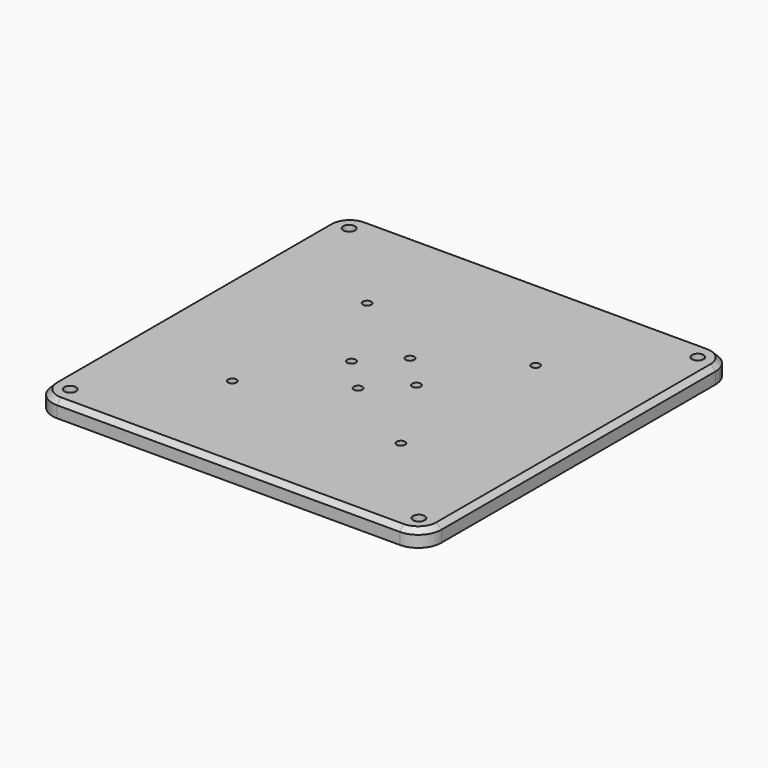
from build123d import *

# Parameters (mm, degrees)
F0_W           = 300
F0_H           = 300
F1_DEPTH       = 12.7
F2_R           = 17.78
F3_SIZE        = 3.81
F5_D           = 9
F7_D           = 6.5278
F9_D           = 6.6
F9_CSINK_D     = 13.44
F9_CSINK_ANGLE = 90


with BuildPart() as f1:
    # F0 (on Top) → F1 (new body)
    with BuildSketch(Plane.XY):
        Rectangle(F0_W, F0_H)
    extrude(amount=F1_DEPTH)

    # F2
    f2_edges = [f1.edges().sort_by_distance(p)[0] for p in [
        (-150, -150, 6.35),
        (150, -150, 6.35),
        (150, 150, 6.35),
        (-150, 150, 6.35),
    ]]
    fillet(f2_edges, radius=F2_R)

    # F3
    f3_edges = [f1.edges().sort_by_distance(p)[0] for p in [
        (-150, 0, 12.7),
        (0, 150, 12.7),
        (150, 0, 12.7),
        (0, -150, 12.7),
        (144.792359, -144.792359, 12.7),
        (144.792359, 144.792359, 12.7),
        (-144.792359, -144.792359, 12.7),
        (-144.792359, 144.792359, 12.7),
    ]]
    chamfer(f3_edges, length=F3_SIZE)

    # F5 (through all)
    with Locations(Plane(origin=(0, 0, 0), x_dir=(1, 0, 0), z_dir=(0, 0, -1))):
        with Locations((-134.5, 134.5), (134.5, 134.5), (-134.5, -134.5), (134.5, -134.5)):
            Hole(F5_D / 2)

    # F7 (through all)
    with Locations(Plane(origin=(0, 0, 0), x_dir=(1, 0, 0), z_dir=(0, 0, -1))):
        with Locations((-65, 65), (65, 65), (65, -65), (-65, -65)):
            Hole(F7_D / 2)

    # F9 (through all)
    with Locations(Plane(origin=(0, 0, 0), x_dir=(1, 0, 0), z_dir=(0, 0, -1))):
        with Locations((0, 25), (25, 0), (0, -25), (-25, 0)):
            CounterSinkHole(F9_D / 2, F9_CSINK_D / 2, counter_sink_angle=F9_CSINK_ANGLE)


solid = f1.part
